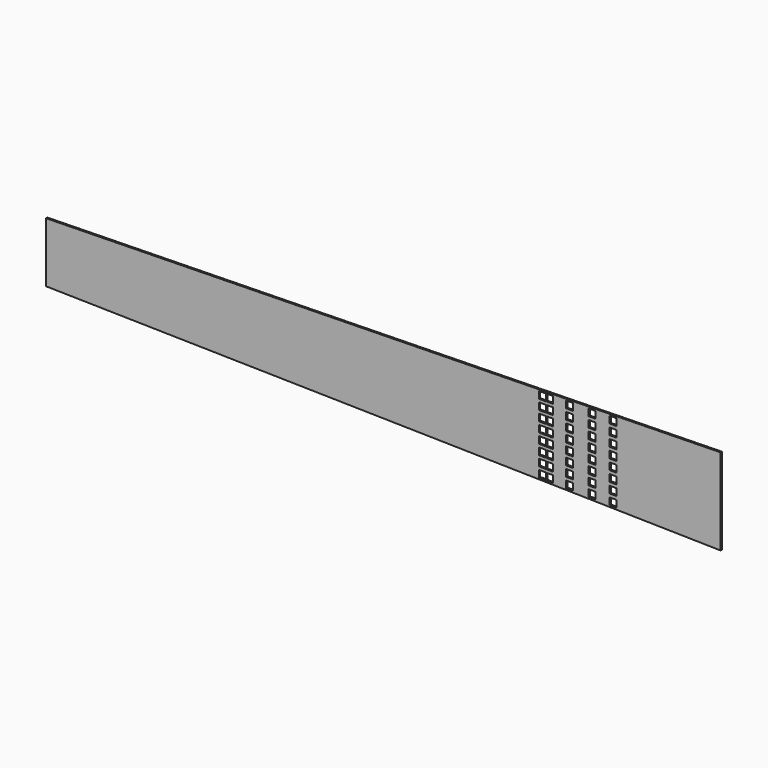
from build123d import *

# Parameters (mm, degrees)
F0_W     = 6.5
F0_H     = 6.5
F1_DEPTH = 1.524
F3_R     = 1.1303
F4_DEPTH = 972


# Not quite as in the source:
# - an extrude ends at something that could not be found from the text; its depth is read off the source's solid


with BuildPart() as f1:
    # F0 (on Front) → F1 (new body)
    with BuildSketch(Plane.XZ):
        Polygon((0, 56.388), (0, 0), (304.8, -5.97408), (304.8, 62.36208), align=None)
        Polygon((304.8, 62.36208), (304.8, -5.97408), (635, -12.446), (635, 68.834), align=None)
        with Locations((467.1477068, -4.4873331716)):
            Rectangle(F0_W, F0_H, mode=Mode.SUBTRACT)
        with Locations((474.1477436, -4.6073838027)):
            Rectangle(F0_W, F0_H, mode=Mode.SUBTRACT)
        with Locations((467.1477068, 4.8497068284)):
            Rectangle(F0_W, F0_H, mode=Mode.SUBTRACT)
        with Locations((474.1477436, 4.7652161973)):
            Rectangle(F0_W, F0_H, mode=Mode.SUBTRACT)
        with Locations((492.8806754, -4.9286535831)):
            Rectangle(F0_W, F0_H, mode=Mode.SUBTRACT)
        with Locations((513.8657236, -5.2885471597)):
            Rectangle(F0_W, F0_H, mode=Mode.SUBTRACT)
        with Locations((533.6728214, -5.628238887)):
            Rectangle(F0_W, F0_H, mode=Mode.SUBTRACT)
        with Locations((492.8806754, 4.5353864169)):
            Rectangle(F0_W, F0_H, mode=Mode.SUBTRACT)
        with Locations((513.8657236, 4.2770928403)):
            Rectangle(F0_W, F0_H, mode=Mode.SUBTRACT)
        with Locations((533.6728214, 4.036461113)):
            Rectangle(F0_W, F0_H, mode=Mode.SUBTRACT)
        with Locations((467.1477068, 14.1867468284)):
            Rectangle(F0_W, F0_H, mode=Mode.SUBTRACT)
        with Locations((474.1477436, 14.1378161973)):
            Rectangle(F0_W, F0_H, mode=Mode.SUBTRACT)
        with Locations((467.1477068, 23.5237868284)):
            Rectangle(F0_W, F0_H, mode=Mode.SUBTRACT)
        with Locations((474.1477436, 23.5104161973)):
            Rectangle(F0_W, F0_H, mode=Mode.SUBTRACT)
        with Locations((492.8806754, 13.9994264169)):
            Rectangle(F0_W, F0_H, mode=Mode.SUBTRACT)
        with Locations((513.8657236, 13.8427328403)):
            Rectangle(F0_W, F0_H, mode=Mode.SUBTRACT)
        with Locations((533.6728214, 13.701161113)):
            Rectangle(F0_W, F0_H, mode=Mode.SUBTRACT)
        with Locations((492.8806754, 23.4634664169)):
            Rectangle(F0_W, F0_H, mode=Mode.SUBTRACT)
        with Locations((513.8657236, 23.4083728403)):
            Rectangle(F0_W, F0_H, mode=Mode.SUBTRACT)
        with Locations((533.6728214, 23.365861113)):
            Rectangle(F0_W, F0_H, mode=Mode.SUBTRACT)
        with Locations((467.1477068, 32.8608268284)):
            Rectangle(F0_W, F0_H, mode=Mode.SUBTRACT)
        with Locations((474.1477436, 32.8830161973)):
            Rectangle(F0_W, F0_H, mode=Mode.SUBTRACT)
        with Locations((467.1477068, 42.1978668284)):
            Rectangle(F0_W, F0_H, mode=Mode.SUBTRACT)
        with Locations((474.1477436, 42.2556161973)):
            Rectangle(F0_W, F0_H, mode=Mode.SUBTRACT)
        with Locations((492.8806754, 32.9275064169)):
            Rectangle(F0_W, F0_H, mode=Mode.SUBTRACT)
        with Locations((513.8657236, 32.9740128403)):
            Rectangle(F0_W, F0_H, mode=Mode.SUBTRACT)
        with Locations((533.6728214, 33.030561113)):
            Rectangle(F0_W, F0_H, mode=Mode.SUBTRACT)
        with Locations((492.8806754, 42.3915464169)):
            Rectangle(F0_W, F0_H, mode=Mode.SUBTRACT)
        with Locations((513.8657236, 42.5396528403)):
            Rectangle(F0_W, F0_H, mode=Mode.SUBTRACT)
        with Locations((533.6728214, 42.695261113)):
            Rectangle(F0_W, F0_H, mode=Mode.SUBTRACT)
        with Locations((467.1477068, 51.5349068284)):
            Rectangle(F0_W, F0_H, mode=Mode.SUBTRACT)
        with Locations((474.1477436, 51.6282161973)):
            Rectangle(F0_W, F0_H, mode=Mode.SUBTRACT)
        with Locations((467.1477068, 60.8719468284)):
            Rectangle(F0_W, F0_H, mode=Mode.SUBTRACT)
        with Locations((474.1477436, 61.0008161973)):
            Rectangle(F0_W, F0_H, mode=Mode.SUBTRACT)
        with Locations((492.8806754, 51.8555864169)):
            Rectangle(F0_W, F0_H, mode=Mode.SUBTRACT)
        with Locations((513.8657236, 52.1052928403)):
            Rectangle(F0_W, F0_H, mode=Mode.SUBTRACT)
        with Locations((533.6728214, 52.359961113)):
            Rectangle(F0_W, F0_H, mode=Mode.SUBTRACT)
        with Locations((492.8806754, 61.3196264169)):
            Rectangle(F0_W, F0_H, mode=Mode.SUBTRACT)
        with Locations((513.8657236, 61.6709328403)):
            Rectangle(F0_W, F0_H, mode=Mode.SUBTRACT)
        with Locations((533.6728214, 62.024661113)):
            Rectangle(F0_W, F0_H, mode=Mode.SUBTRACT)
    extrude(amount=F1_DEPTH)

    # F3 (on face) → F4 (cut, through all)
    with BuildSketch(Plane.XZ.offset(1.524)):
        with Locations((97.3946236, 8.0847413075)):
            Circle(F3_R)
        with Locations((3.175, 8.1216754)):
            Circle(F3_R)
        with Locations((181.3279076, 8.0518394602)):
            Circle(F3_R)
        with Locations((290.391088, 8.0090866935)):
            Circle(F3_R)
        with Locations((409.2984448, 7.9624750096)):
            Circle(F3_R)
        with Locations((524.05534, 7.9174903067)):
            Circle(F3_R)
        with Locations((624.435886, 7.8781411327)):
            Circle(F3_R)
        with Locations((97.3946236, 48.3032586925)):
            Circle(F3_R)
        with Locations((3.175, 48.2663246)):
            Circle(F3_R)
        with Locations((181.3279076, 48.3361605398)):
            Circle(F3_R)
        with Locations((290.391088, 48.3789133065)):
            Circle(F3_R)
        with Locations((409.2984448, 48.4255249904)):
            Circle(F3_R)
        with Locations((524.05534, 48.4705096933)):
            Circle(F3_R)
        with Locations((624.435886, 48.5098588673)):
            Circle(F3_R)
    extrude(amount=F4_DEPTH, mode=Mode.SUBTRACT)


solid = f1.part
